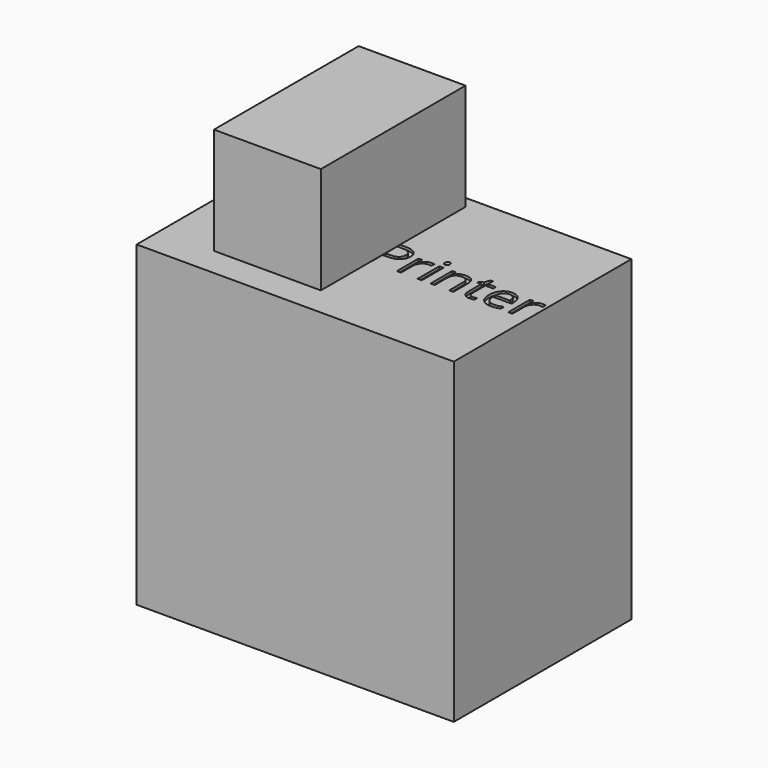
from build123d import *

# Parameters (mm, degrees)
F0_W         = 762
F0_H         = 533.4
F1_DEPTH     = 762
F2_W         = 256.9460421801
F2_H         = 434.4925582409
F3_DEPTH     = 256.54
F4_TEXT_SIZE = 122.1938886576
F5_DEPTH     = 6.35
F6_DEPTH     = 6.35


# Not quite as in the source:
# - Text() gives the source's letters only with a copy of the font that has no kerning and outlines rounded to 1/6400 em; it was checked with that copy


with BuildPart() as f1:
    # F0 (on Top) → F1 (new body)
    with BuildSketch(Plane.XY):
        with Locations((381, 266.7)):
            Rectangle(F0_W, F0_H)
    extrude(amount=F1_DEPTH)

    # F2 (on face) → F3 (join)
    with BuildSketch(Plane.XY.offset(762)):
        with Locations((258.0651268363, 287.4724417925)):
            Rectangle(F2_W, F2_H)
    extrude(amount=F3_DEPTH)

    # F4 (on face) → F5 (cut)
    with BuildSketch(Plane.XY.offset(762)):
        with Locations((364.8698618627, 220.5050885677)):
            Text('Printer', F4_TEXT_SIZE, font='Open Sans', text_align=(TextAlign.LEFT, TextAlign.BOTTOM))
    extrude(amount=-F5_DEPTH, mode=Mode.SUBTRACT)

    # F4 (on face) → F6 (cut)
    with BuildSketch(Plane.XY.offset(762)):
        with Locations((364.8698618627, 220.5050885677)):
            Text('Printer', F4_TEXT_SIZE, font='Open Sans', text_align=(TextAlign.LEFT, TextAlign.BOTTOM))
    extrude(amount=-F6_DEPTH, mode=Mode.SUBTRACT)


solid = f1.part
